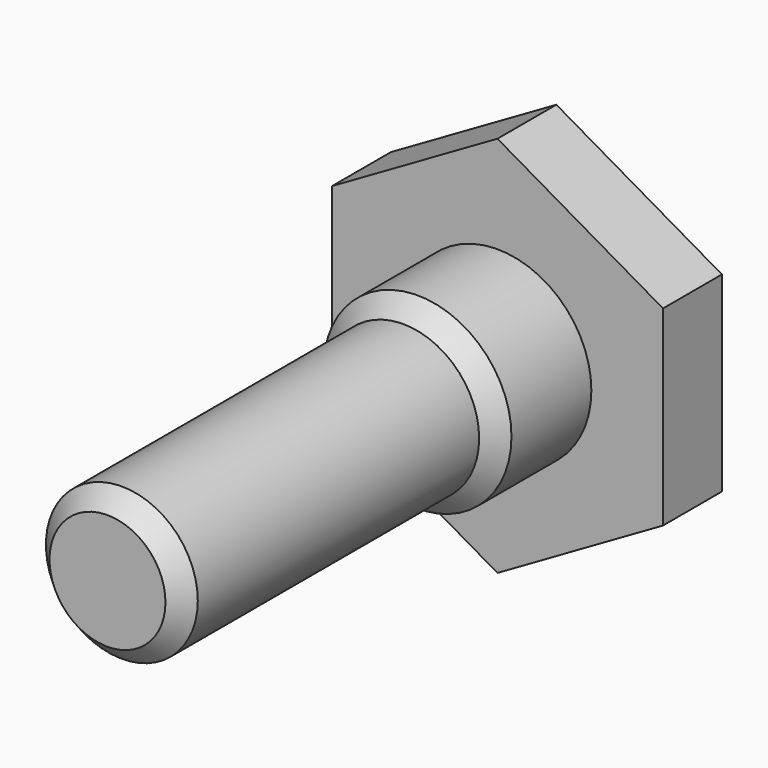
from build123d import *

# Parameters (mm, degrees)
F1_DEPTH = 20.5
F2_R     = 26.136981888
F3_DEPTH = 32.8
F4_SIZE  = 5
F5_DEPTH = 102.9
F6_SIZE  = 5


with BuildPart() as f1:
    # F0 (on Front) → F1 (new body)
    with BuildSketch(Plane.XZ):
        Polygon((46.0798591375, -26.6042190773), (46.0798591375, 26.6042190773), (0, 53.2084381546), (-46.0798591375, 26.6042190773), (-46.0798591375, -26.6042190773), (0, -53.2084381546), align=None)
    extrude(amount=F1_DEPTH)

    # F2 (on face) → F3 (join)
    with BuildSketch(Plane.XZ.offset(20.5)):
        Circle(F2_R)
    extrude(amount=F3_DEPTH)

    # F4
    f4_edges = [f1.edges().sort_by_distance(p)[0] for p in [
        (-26.136982, -53.3, 0),
    ]]
    chamfer(f4_edges, length=F4_SIZE)

    # F5 (add): a face of the model
    f5_faces = [f1.faces().sort_by_distance(p)[0] for p in [
        (0, -53.3, 0),
    ]]
    extrude(f5_faces, amount=F5_DEPTH)

    # F6
    f6_edges = [f1.edges().sort_by_distance(p)[0] for p in [
        (-21.136982, -156.2, 0),
    ]]
    chamfer(f6_edges, length=F6_SIZE)


solid = f1.part
